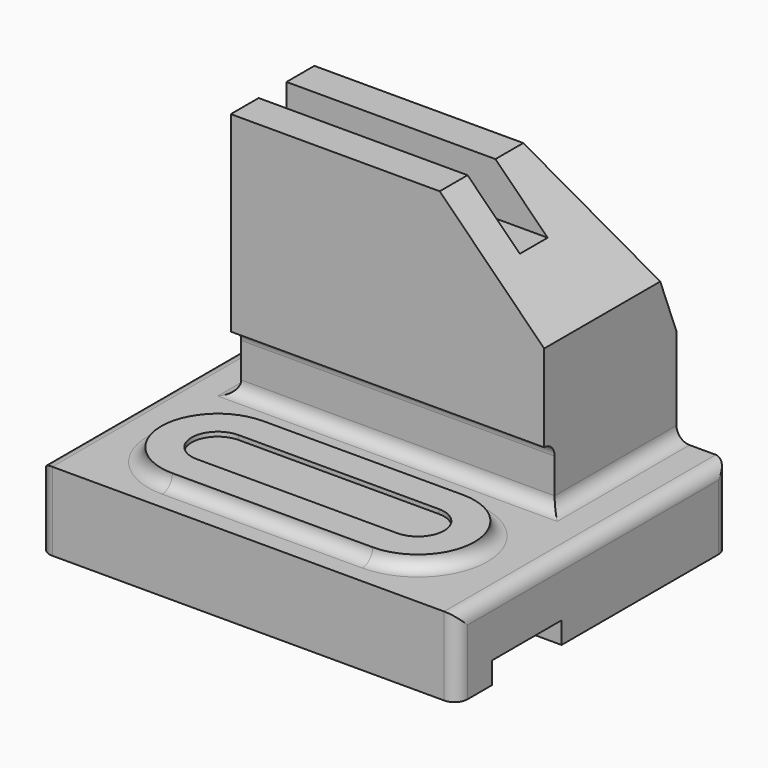
from build123d import *

# Parameters (mm, degrees)
F0_W      = 96
F0_H      = 78
F1_DEPTH  = 18
F3_W      = 72
F3_H      = 38
F5_DEPTH  = 58
F7_DEPTH  = 38
F8_W      = 8
F8_H      = 12
F9_DEPTH  = 60.001
F11_DEPTH = 72.001
F12_W     = 20
F12_H     = 5
F13_DEPTH = 96.001
F14_W     = 46
F14_H     = 26
F15_DEPTH = 3
F16_W     = 46
F16_H     = 12
F17_DEPTH = 1
F18_W     = 3
F18_H     = 14
F19_DEPTH = 72
F20_R     = 2.99999


# Not quite as in the source:
# - a fillet or chamfer is up to 0.001 mm smaller than in the source, because OpenCascade refuses the exact size


with BuildPart() as f1:
    # F0 (on Top) → F1 (new body)
    with BuildSketch(Plane.XY):
        with Locations((48, 39)):
            Rectangle(F0_W, F0_H)
    extrude(amount=F1_DEPTH)

    # F3 (on face) → F5 (join, through all)
    with BuildSketch(Plane.XY.offset(18)):
        with Locations((48, 59)):
            Rectangle(F3_W, F3_H)
    extrude(amount=F5_DEPTH)

    # F6 (on face) → F7 (cut, through all)
    with BuildSketch(Plane.XZ.offset(-40)):
        Polygon((84, 76), (60, 76), (84, 52), align=None)
    extrude(amount=-F7_DEPTH, mode=Mode.SUBTRACT)

    # F8 (on face) → F9 (cut, through all)
    with BuildSketch(Plane(origin=(12, 0, 0), x_dir=(0, -1, 0), z_dir=(-1, 0, 0))):
        with Locations((-52, 70)):
            Rectangle(F8_W, F8_H)
    extrude(amount=-F9_DEPTH, mode=Mode.SUBTRACT)

    # F10 (on face) → F11 (cut, through all)
    with BuildSketch(Plane(origin=(12, 0, 0), x_dir=(0, -1, 0), z_dir=(-1, 0, 0))):
        Polygon((-64, 76), (-78, 76), (-78, 40), align=None)
    extrude(amount=-F11_DEPTH, mode=Mode.SUBTRACT)

    # F12 (on face) → F13 (cut, through all)
    with BuildSketch(Plane.YZ.offset(96)):
        with Locations((20, 2.5)):
            Rectangle(F12_W, F12_H)
    extrude(amount=-F13_DEPTH, mode=Mode.SUBTRACT)

    # F14 (on face) → F15 (join)
    with BuildSketch(Plane.XY.offset(18)):
        with Locations((48, 19.9999999999)):
            Rectangle(F14_W, F14_H)
        with BuildLine():
            Line((25, 6.9999999999), (25, 32.9999999999))
            ThreePointArc((25, 32.9999999999), (12, 19.9999999999), (25, 6.9999999999))
        make_face()
        with BuildLine():
            ThreePointArc((71, 6.9999999999), (84, 19.9999999999), (71, 32.9999999999))
            Line((71, 32.9999999999), (71, 6.9999999999))
        make_face()
    extrude(amount=F15_DEPTH)

    # F16 (on face) → F17 (cut, through all)
    with BuildSketch(Plane.XY.offset(21)):
        with Locations((48, 19.9999999999)):
            Rectangle(F16_W, F16_H)
        with BuildLine():
            Line((25, 13.9999999999), (25, 25.9999999999))
            ThreePointArc((25, 25.9999999999), (19, 19.9999999999), (25, 13.9999999999))
        make_face()
        with BuildLine():
            ThreePointArc((71, 13.9999999999), (77, 19.9999999999), (71, 25.9999999999))
            Line((71, 25.9999999999), (71, 13.9999999999))
        make_face()
    extrude(amount=-F17_DEPTH, mode=Mode.SUBTRACT)

    # F18 (on face) → F19 (cut, through all)
    with BuildSketch(Plane.YZ.offset(84)):
        with Locations((41.5, 25)):
            Rectangle(F18_W, F18_H)
    extrude(amount=-F19_DEPTH, mode=Mode.SUBTRACT)

    # F20 (radius 3 in the source; OpenCascade refuses exactly that, so slightly less here)
    f20_edges = [f1.edges().sort_by_distance(p)[0] for p in [
        (48, 43, 32),
        (48, 43, 18),
        (48, 33, 18),
        (48, 7, 18),
        (96, 39, 18),
        (0, 39, 18),
        (84, 60.5, 18),
        (12, 60.5, 18),
        (96, 0, 9),
        (0, 0, 9),
        (0, 78, 9),
        (96, 78, 9),
    ]]
    fillet(f20_edges, radius=F20_R)


solid = f1.part
